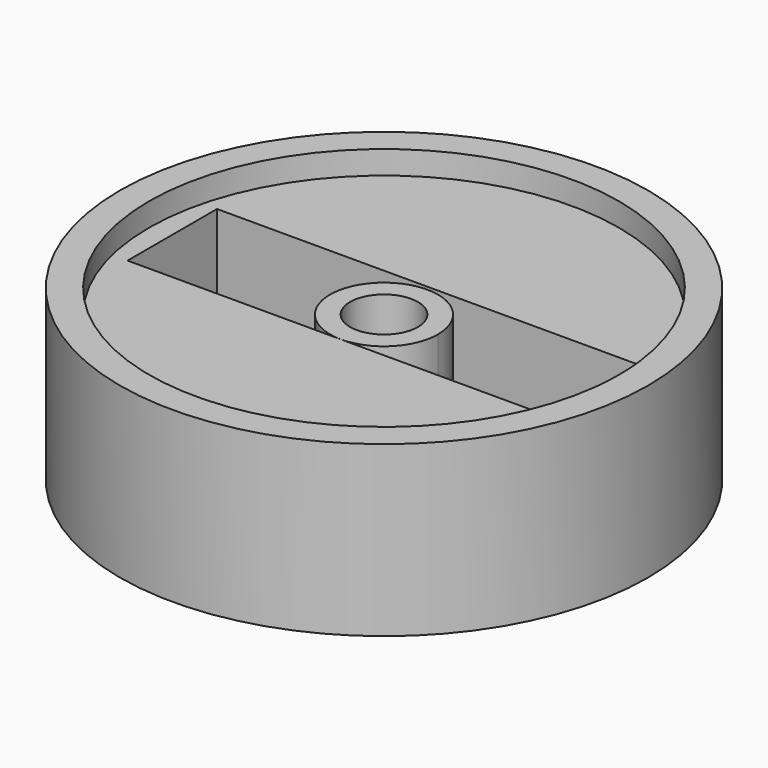
from build123d import *

# Parameters (mm, degrees)
F0_R     = 45.3102610886
F1_DEPTH = 29
F2_DEPTH = 30
F0_R_2   = 5.8189451516
F3_DEPTH = 25


with BuildPart() as f1:
    # F0 (on Top) → F1 (new body)
    with BuildSketch(Plane.XY):
        with Locations((0, 4.6897389114)):
            Circle(F0_R)
        with BuildLine():
            ThreePointArc((40.0365270468, 0), (-5.2843801511, -35.2726493486), (-39.8794180788, 10.567592493))
            ThreePointArc((-39.8794180788, 10.567592493), (0.5992286077, 44.9955458641), (40.0365270468, 9.3794778229))
            ThreePointArc((40.0365270468, 9.3794778229), (40.2417693905, 7.038599347), (40.3102610886, 4.6897389114))
            ThreePointArc((40.3102610886, 4.6897389114), (40.2417693905, 2.3408784759), (40.0365270468, 0))
        make_face(mode=Mode.SUBTRACT)
    extrude(amount=F1_DEPTH)

    # F0 (on Top) → F2 (cut)
    with BuildSketch(Plane.XY):
        with Locations((0, 4.6897389114)):
            Circle(F0_R)
        with BuildLine():
            ThreePointArc((40.0365270468, 0), (-5.2843801511, -35.2726493486), (-39.8794180788, 10.567592493))
            ThreePointArc((-39.8794180788, 10.567592493), (0.5992286077, 44.9955458641), (40.0365270468, 9.3794778229))
            ThreePointArc((40.0365270468, 9.3794778229), (40.2417693905, 7.038599347), (40.3102610886, 4.6897389114))
            ThreePointArc((40.3102610886, 4.6897389114), (40.2417693905, 2.3408784759), (40.0365270468, 0))
        make_face(mode=Mode.SUBTRACT)
    extrude(amount=-F2_DEPTH, mode=Mode.SUBTRACT)



with BuildPart() as f3:
    # F0 (on Top) → F3 (new body)
    with BuildSketch(Plane.XY):
        with BuildLine():
            ThreePointArc((0, -4.5645707527), (6.5437851187, -1.8540462073), (9.2543096641, 4.6897389114))
            ThreePointArc((9.2543096641, 4.6897389114), (-6.5437851187, 11.2335240302), (0, -4.5645707527))
        make_face()
        with Locations((0, 4.6897389114)):
            Circle(F0_R_2, mode=Mode.SUBTRACT)
    extrude(amount=F3_DEPTH)


with BuildPart() as f1_1:
    add(f1.part)

    add(f3.part)  # F3#2 merges F3
    # F0 (on Top) → F3, piece 2 (join)
    with BuildSketch(Plane.XY):
        with BuildLine():
            ThreePointArc((40.0365270468, 9.3794778229), (0.5992286077, 44.9955458641), (-39.8794180788, 10.567592493))
            ThreePointArc((-39.8794180788, 10.567592493), (-5.2843801511, -35.2726493486), (40.0365270468, 0))
            Line((40.0365270468, 0), (40.0365270468, 9.3794778229))
        make_face()
        Polygon((35.6006100774, -4.5645707527), (0, -4.5645707527), (-36.5868918598, -4.5645707527), (-36.5868918598, 14.6164782345), (35.6006100774, 14.6164782345), align=None, mode=Mode.SUBTRACT)
    extrude(amount=F3_DEPTH)


solid = f1_1.part
